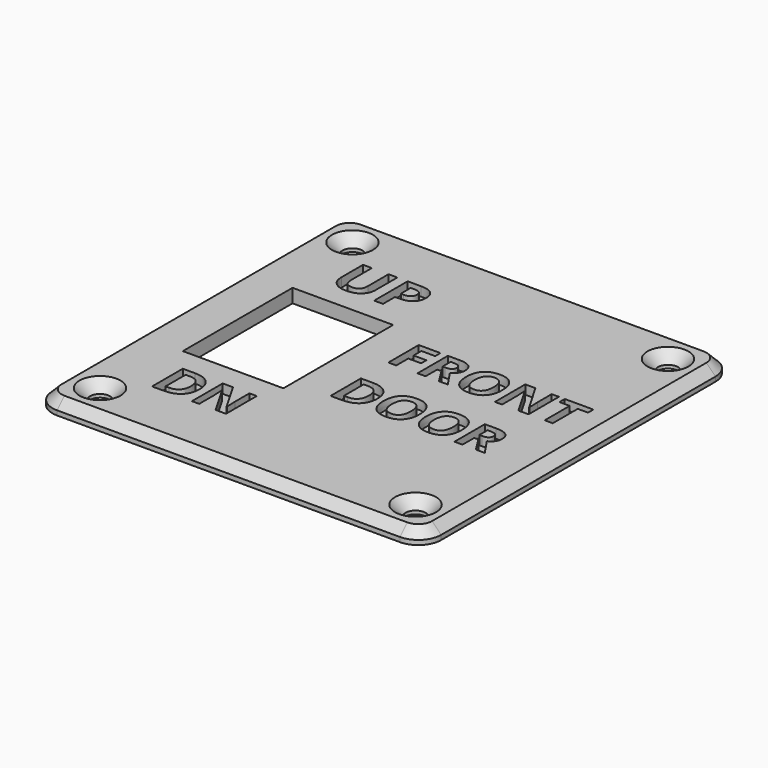
from build123d import *

# Parameters (mm, degrees)
F0_R           = 2
F0_W           = 22
F0_H           = 30
F0_W_2         = 27.5
F0_H_2         = 33
F1_DEPTH       = 3
F0_W_3         = 21.5
F0_H_3         = 27
F2_DEPTH       = 10
F2_DEPTH_BACK  = 3
F3_DEPTH       = 3
F4_SIZE        = 2
F5_TEXT_SIZE   = 12.8227960819
F5_TEXT_SIZE_2 = 11.7779368163
F5_TEXT_SIZE_3 = 11.621572544
F6_DEPTH       = 2
F8_D           = 4.4
F8_CSINK_D     = 8.96
F8_CSINK_ANGLE = 90


# Not quite as in the source:
# - Text() gives the source's letters only with a copy of the font that has no kerning and outlines rounded to 1/6400 em; it was checked with that copy


with BuildPart() as f1:
    # F0 (on Top) → F1 (new body)
    with BuildSketch(Plane.XY):
        with BuildLine():
            Line((37.5, 42.5), (-37.5, 42.5))
            ThreePointArc((-37.5, 42.5), (-41.0355339059, 41.0355339059), (-42.5, 37.5))
            Line((-42.5, 37.5), (-42.5, -37.5))
            ThreePointArc((-42.5, -37.5), (-41.0355339059, -41.0355339059), (-37.5, -42.5))
            Line((-37.5, -42.5), (37.5, -42.5))
            ThreePointArc((37.5, -42.5), (41.0355339059, -41.0355339059), (42.5, -37.5))
            Line((42.5, -37.5), (42.5, 37.5))
            ThreePointArc((42.5, 37.5), (41.0355339059, 41.0355339059), (37.5, 42.5))
        make_face()
        with Locations((-34.5, -34.5)):
            Circle(F0_R, mode=Mode.SUBTRACT)
        with Locations((34.5, -34.5)):
            Circle(F0_R, mode=Mode.SUBTRACT)
        with Locations((-21, 0)):
            Rectangle(F0_W, F0_H, mode=Mode.SUBTRACT)
        with Locations((-34.5, 34.5)):
            Circle(F0_R, mode=Mode.SUBTRACT)
        with Locations((13.75, 0)):
            Rectangle(F0_W_2, F0_H_2, mode=Mode.SUBTRACT)
        with Locations((34.5, 34.5)):
            Circle(F0_R, mode=Mode.SUBTRACT)
    extrude(amount=F1_DEPTH)

    # F0 (on Top) → F2 (join, two sides)
    with BuildSketch(Plane.XY) as f2_sk:
        with Locations((13.75, 0)):
            Rectangle(F0_W_2, F0_H_2)
        with Locations((13.75, 0)):
            Rectangle(F0_W_3, F0_H_3, mode=Mode.SUBTRACT)
    extrude(amount=-F2_DEPTH)
    extrude(f2_sk.sketch, amount=F2_DEPTH_BACK)

    # F0 (on Top) → F3 (join)
    with BuildSketch(Plane.XY):
        with Locations((13.75, 0)):
            Rectangle(F0_W_3, F0_H_3)
    extrude(amount=F3_DEPTH)

    # F4
    f4_edges = [f1.edges().sort_by_distance(p)[0] for p in [
        (0, -42.5, 3),
    ]]
    chamfer(f4_edges, length=F4_SIZE)

    # F5 (on face) → F6 (cut)
    with BuildSketch(Plane.XY.offset(3)):
        with Locations((-29, 20)):
            Text('UP', F5_TEXT_SIZE, font='Open Sans', font_style=FontStyle.BOLD, text_align=(TextAlign.LEFT, TextAlign.BOTTOM))
        with Locations((-29, -28.4801145077)):
            Text('DN', F5_TEXT_SIZE_2, font='Open Sans', font_style=FontStyle.BOLD, text_align=(TextAlign.LEFT, TextAlign.BOTTOM))
        with Locations((-3, 3.6324677683)):
            Text('FRONT', F5_TEXT_SIZE_3, font='Open Sans', font_style=FontStyle.BOLD, text_align=(TextAlign.LEFT, TextAlign.BOTTOM))
        with Locations((-3, -12.1728708916)):
            Text('DOOR', F5_TEXT_SIZE_3, font='Open Sans', font_style=FontStyle.BOLD, text_align=(TextAlign.LEFT, TextAlign.BOTTOM))
    extrude(amount=-F6_DEPTH, mode=Mode.SUBTRACT)

    # F8 (through all)
    with Locations(Plane.XY.offset(3)):
        with Locations((-34.5, 34.5), (34.5, 34.5), (34.5, -34.5), (-34.5, -34.5)):
            CounterSinkHole(F8_D / 2, F8_CSINK_D / 2, counter_sink_angle=F8_CSINK_ANGLE)


solid = f1.part
